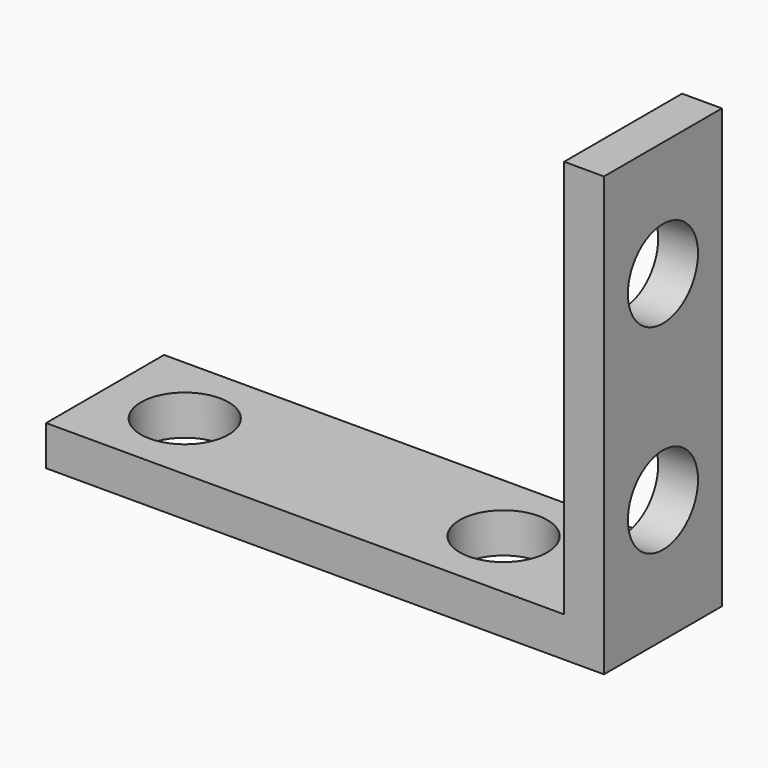
from build123d import *

# Parameters (mm, degrees)
F0_W     = 28
F0_H     = 7.4
F1_DEPTH = 22
F3_D     = 4.4
F4_W     = 26
F4_H     = 20
F5_DEPTH = 25
F7_D     = 4.4


# Not quite as in the source:
# - a feature of the source that left no trace in its solid (it failed there, or was rolled back) is left out
# - a feature names something its author has since deleted; it is built from what else it names


with BuildPart() as f1:
    # F0 (on Top) → F1 (new body)
    with BuildSketch(Plane.XY):
        with Locations((-14, -3.7)):
            Rectangle(F0_W, F0_H)
    extrude(amount=F1_DEPTH)

    # F3 (through all)
    with Locations(Plane.XY.offset(22)):
        with Locations((-24, -3.7), (-8, -3.7)):
            Hole(F3_D / 2)

    # F4 (on face) → F5 (cut)
    with BuildSketch(Plane(origin=(0, 0, 0), x_dir=(-1, 0, 0), z_dir=(0, 1, 0))):
        with Locations((15, 12)):
            Rectangle(F4_W, F4_H)
    extrude(amount=-F5_DEPTH, mode=Mode.SUBTRACT)

    # F7 (through all)
    with Locations(Plane(origin=(-2, 0, 0), x_dir=(0, -1, 0), z_dir=(-1, 0, 0))):
        with Locations((3.7, 16.2), (3.7, 6.2)):
            Hole(F7_D / 2)


solid = f1.part
